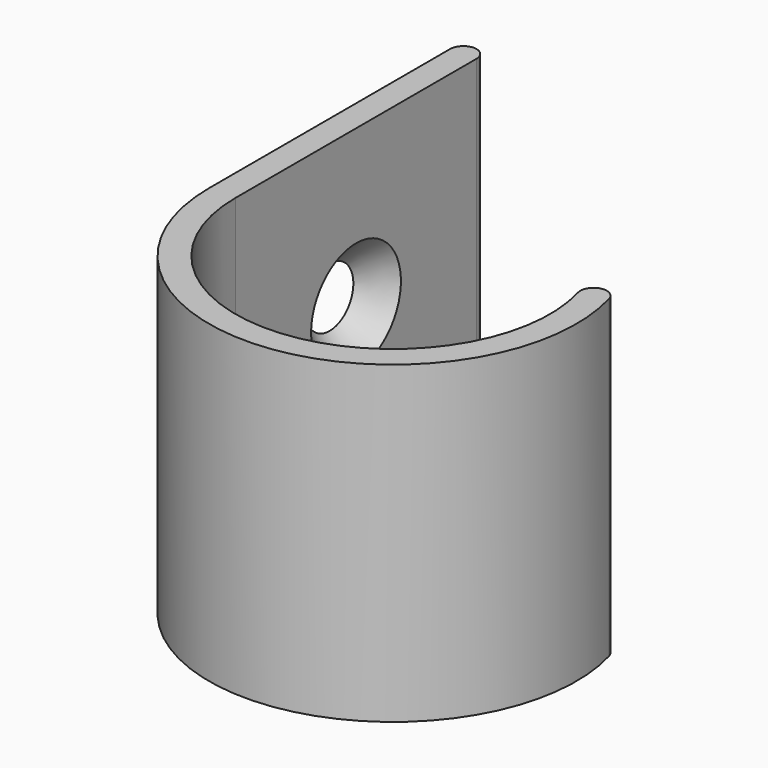
from build123d import *

# Parameters (mm, degrees)
F1_DEPTH       = 19.05
F2_R           = 0.79999
F4_D           = 3.4
F4_CSINK_D     = 6.8
F4_CSINK_ANGLE = 90


# Not quite as in the source:
# - a fillet or chamfer is up to 0.001 mm smaller than in the source, because OpenCascade refuses the exact size


with BuildPart() as f1:
    # F0 (on Top) → F1 (new body)
    with BuildSketch(Plane.XY):
        with BuildLine():
            ThreePointArc((18.475572213, 3.2577418652), (11.1789988923, -9.3802938474), (0, 0))
            Line((0, 0), (0, 18.25))
            ThreePointArc((0, 18.25), (-0.2343145751, 18.8156854249), (-0.8, 19.05))
            ThreePointArc((-0.8, 19.05), (-1.3656854249, 18.8156854249), (-1.6, 18.25))
            Line((-1.6, 18.25), (-1.6, 0))
            ThreePointArc((-1.6, 0), (11.4568359765, -10.9559862523), (19.9790804062, 3.8049740945))
            Line((19.9790804062, 3.8049740945), (18.475572213, 3.2577418652))
        make_face()
    extrude(amount=F1_DEPTH)

    # F2 (radius 0.8 in the source; OpenCascade refuses exactly that, so slightly less here)
    f2_edges = [f1.edges().sort_by_distance(p)[0] for p in [
        (19.97908, 3.804974, 9.525),
        (18.475572, 3.257742, 9.525),
    ]]
    fillet(f2_edges, radius=F2_R)

    # F4 (through all)
    with Locations(Plane.YZ):
        with Locations((9.125, 9.525)):
            CounterSinkHole(F4_D / 2, F4_CSINK_D / 2, counter_sink_angle=F4_CSINK_ANGLE)


solid = f1.part
